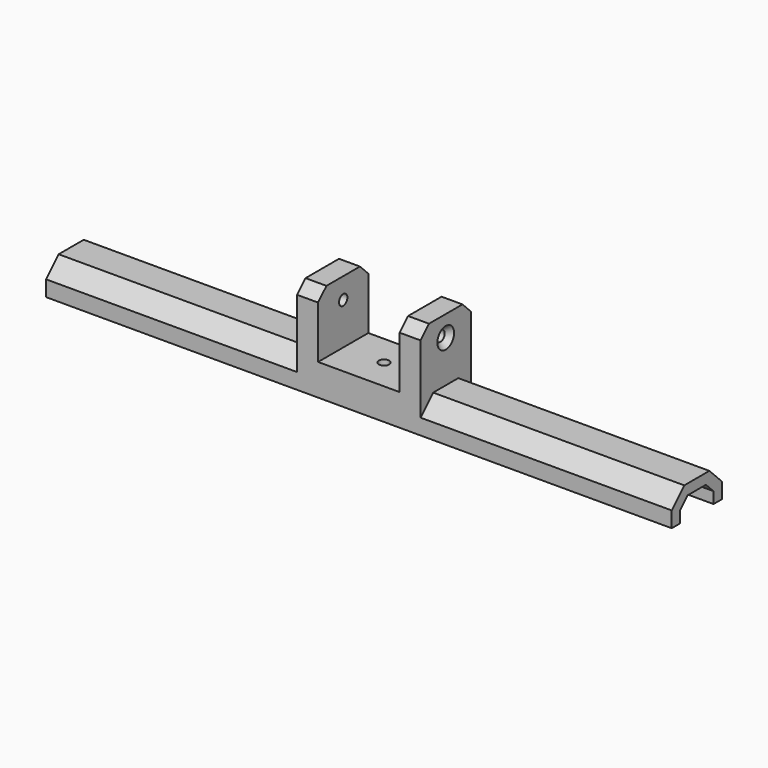
from build123d import *

# Parameters (mm, degrees)
F1_DEPTH = 30
F2_SIZE  = 7.5
F4_DEPTH = 299.001
F5_SIZE  = 5
F6_R     = 2.5
F7_DEPTH = 179.001
F8_R     = 2.5
F9_DEPTH = 15.001
F10_SIZE = 2.5


with BuildPart() as f1:
    # F0 (on Front) → F1 (new body)
    with BuildSketch(Plane.XZ):
        Polygon((-149.5, 0), (0, 0), (149.5, 0), (149.5, 15), (29.5, 15), (29.5, 45), (19.5, 45), (19.5, 15), (0, 15), (-19.5, 15), (-19.5, 45), (-29.5, 45), (-29.5, 15), (-149.5, 15), align=None)
    extrude(amount=F1_DEPTH)

    # F2
    f2_edges = [f1.edges().sort_by_distance(p)[0] for p in [
        (-89.5, -30, 15),
        (-89.5, 0, 15),
        (89.5, 0, 15),
        (89.5, -30, 15),
    ]]
    chamfer(f2_edges, length=F2_SIZE)

    # F3 (on face) → F4 (cut, through all)
    with BuildSketch(Plane(origin=(-149.5, 0, 0), x_dir=(0, -1, 0), z_dir=(-1, 0, 0))):
        Polygon((5.000000033, 5.4289321745), (5.000000033, 0), (24.999999967, 0), (24.999999967, 5.4289321745), (20.4289321745, 9.999999967), (9.5710678255, 9.999999967), align=None)
    extrude(amount=-F4_DEPTH, mode=Mode.SUBTRACT)

    # F5
    f5_edges = [f1.edges().sort_by_distance(p)[0] for p in [
        (-24.5, 0, 45),
        (-24.5, -30, 45),
        (24.5, 0, 45),
        (24.5, -30, 45),
    ]]
    chamfer(f5_edges, length=F5_SIZE)

    # F6 (on face) → F7 (cut, through all)
    with BuildSketch(Plane.YZ.offset(29.5)):
        with Locations((-15, 35)):
            Circle(F6_R)
    extrude(amount=-F7_DEPTH, mode=Mode.SUBTRACT)

    # F8 (on face) → F9 (cut, through all)
    with BuildSketch(Plane.XY.offset(15)):
        with Locations((0, -15)):
            Circle(F8_R)
    extrude(amount=-F9_DEPTH, mode=Mode.SUBTRACT)

    # F10
    f10_edges = [f1.edges().sort_by_distance(p)[0] for p in [
        (-29.5, -17.5, 35),
        (29.5, -17.5, 35),
        (-2.5, -15, 10),
    ]]
    chamfer(f10_edges, length=F10_SIZE)


solid = f1.part
